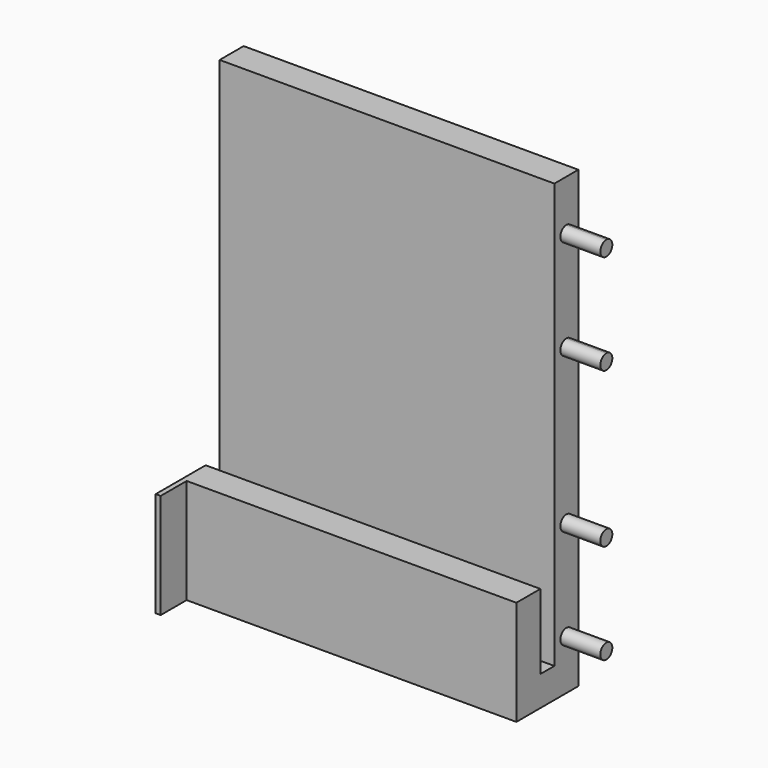
from build123d import *

# Parameters (mm, degrees)
F1_DEPTH  = 67
F2_R      = 1.5
F3_DEPTH  = 8
F4_R      = 1.875
F5_DEPTH  = 9
F6_R      = 1.875
F7_DEPTH  = 9
F8_W      = 1
F8_H      = 21
F9_DEPTH  = 6.5
F10_R     = 1.875
F11_DEPTH = 9


# Not quite as in the source:
# - a feature names something its author has since deleted; it is built from what else it names


with BuildPart() as f1:
    # F0 (on Right) → F1 (new body)
    with BuildSketch(Plane.YZ):
        Polygon((14.9777059274, -37.1211464703), (14.9777059274, 53.8788535297), (8.9777059274, 53.8788535297), (8.9777059274, -31.1211464703), (5.4777059274, -31.1211464703), (5.4777059274, -16.1211464703), (-0.5222940726, -16.1211464703), (-0.5222940726, -37.1211464703), align=None)
    extrude(amount=F1_DEPTH)

    # F2 (on face) → F3 (join)
    with BuildSketch(Plane.YZ.offset(67)):
        with BuildLine():
            Line((11.9777059274, 43.8788535297), (11.9777059274, 45.3788535297))
            ThreePointArc((11.9777059274, 45.3788535297), (10.4777059274, 43.8788535297), (11.9777059274, 42.3788535297))
            Line((11.9777059274, 42.3788535297), (11.9777059274, 43.8788535297))
        make_face()
        with BuildLine():
            ThreePointArc((11.9777059274, 42.3788535297), (13.0383660992, 42.8181933579), (13.4777059274, 43.8788535297))
            ThreePointArc((13.4777059274, 43.8788535297), (13.0383660992, 44.9395137015), (11.9777059274, 45.3788535297))
            Line((11.9777059274, 45.3788535297), (11.9777059274, 43.8788535297))
            Line((11.9777059274, 43.8788535297), (11.9777059274, 42.3788535297))
        make_face()
        with BuildLine():
            ThreePointArc((13.4777059274, 23.8788535297), (13.0383660992, 24.9395137015), (11.9777059274, 25.3788535297))
            ThreePointArc((11.9777059274, 25.3788535297), (10.9170457557, 22.8181933579), (13.4777059274, 23.8788535297))
        make_face()
        with Locations((11.9777059274, -7.1211464703)):
            Circle(F2_R)
        with Locations((11.9777059274, -27.1211464703)):
            Circle(F2_R)
    extrude(amount=F3_DEPTH)

    # F4 (on face) → F5 (cut)
    with BuildSketch(Plane(origin=(0, 0, 0), x_dir=(0, -1, 0), z_dir=(-1, 0, 0))):
        with Locations((-18.4777059274, 23.8788535297)):
            Circle(F4_R)
        with Locations((-18.4777059274, 43.8788535297)):
            Circle(F4_R)
        with Locations((-18.4777059274, -7.1211464703)):
            Circle(F4_R)
        with Locations((-18.4777059274, -27.1211464703)):
            Circle(F4_R)
    extrude(amount=-F5_DEPTH, mode=Mode.SUBTRACT)

    # F6 (on face) → F7 (cut)
    with BuildSketch(Plane(origin=(0, 14.9777059274, 0), x_dir=(-1, 0, 0), z_dir=(0, 1, 0))):
        with Locations((-47, -34.1211464703)):
            Circle(F6_R)
        with Locations((-20, -34.1211464703)):
            Circle(F6_R)
    extrude(amount=-F7_DEPTH, mode=Mode.SUBTRACT)

    # F8 (on face) → F9 (join)
    with BuildSketch(Plane.XZ.offset(0.5222940726)):
        with Locations((0.5, -26.6211464703)):
            Rectangle(F8_W, F8_H)
    extrude(amount=F9_DEPTH)

    # F10 (on face) → F11 (cut)
    with BuildSketch(Plane(origin=(0, 0, 0), x_dir=(0, -1, 0), z_dir=(-1, 0, 0))):
        with BuildLine():
            ThreePointArc((-10.1027059274, 43.8788535297), (-10.6518807127, 45.2046787444), (-11.9777059274, 45.7538535297))
            Line((-11.9777059274, 45.7538535297), (-11.9777059274, 43.8788535297))
            Line((-11.9777059274, 43.8788535297), (-11.9777059274, 42.0038535297))
            ThreePointArc((-11.9777059274, 42.0038535297), (-10.6518807127, 42.553028315), (-10.1027059274, 43.8788535297))
        make_face()
        with BuildLine():
            ThreePointArc((-10.1027059274, 23.8788535297), (-10.6518807127, 25.2046787444), (-11.9777059274, 25.7538535297))
            ThreePointArc((-11.9777059274, 25.7538535297), (-13.3035311422, 22.553028315), (-10.1027059274, 23.8788535297))
        make_face()
        with BuildLine():
            Line((-11.9777059274, 43.8788535297), (-11.9777059274, 45.7538535297))
            ThreePointArc((-11.9777059274, 45.7538535297), (-13.8527059274, 43.8788535297), (-11.9777059274, 42.0038535297))
            Line((-11.9777059274, 42.0038535297), (-11.9777059274, 43.8788535297))
        make_face()
        with Locations((-11.9777059274, -27.1211464703)):
            Circle(F10_R)
        with Locations((-11.9777059274, -7.1211464703)):
            Circle(F10_R)
    extrude(amount=-F11_DEPTH, mode=Mode.SUBTRACT)


solid = f1.part
